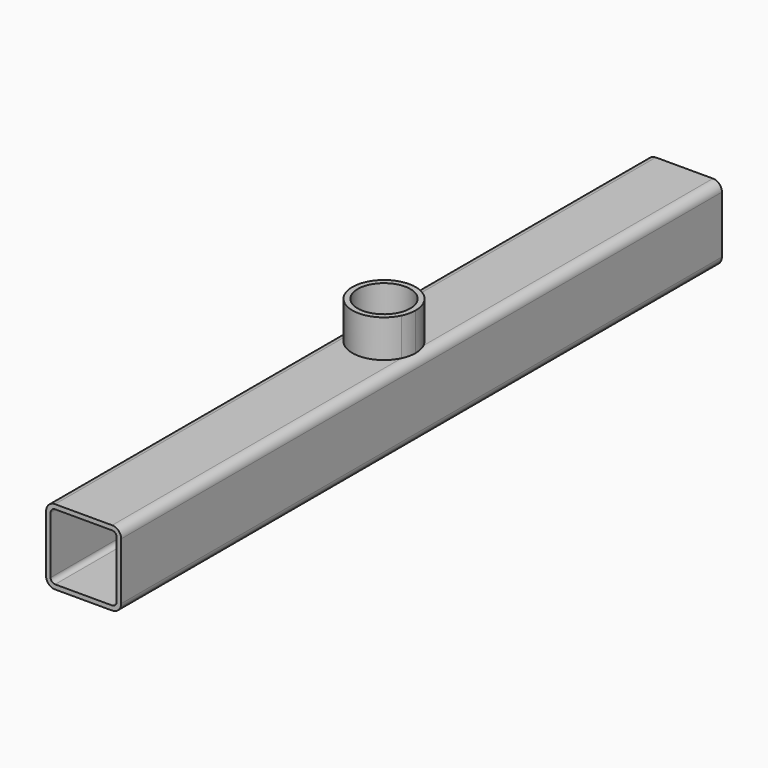
from build123d import *

# Parameters (mm, degrees)
F0_W     = 50
F0_H     = 50
F1_DEPTH = 500
F2_R     = 6
F3_T     = -3
F4_R     = 17.526
F5_DEPTH = 25


with BuildPart() as f1:
    # F0 (on Front) → F1 (new body)
    with BuildSketch(Plane.XZ):
        Rectangle(F0_W, F0_H)
    extrude(amount=F1_DEPTH)

    # F2
    f2_edges = [f1.edges().sort_by_distance(p)[0] for p in [
        (25, -250, 25),
        (-25, -250, 25),
        (25, -250, -25),
        (-25, -250, -25),
    ]]
    fillet(f2_edges, radius=F2_R)

    # F3
    f3_openings = [f1.faces().sort_by_distance(p)[0] for p in [
        (0, 0, 0),
        (0, -500, 0),
    ]]
    offset(amount=F3_T, openings=f3_openings)

    # F4 (on face) → F5 (join)
    with BuildSketch(Plane.XY.offset(25)):
        with BuildLine():
            ThreePointArc((19, -259.1351367806), (20.5549108974, -254.6846944404), (21.082, -250))
            ThreePointArc((21.082, -250), (20.5549108974, -245.3153055596), (19, -240.8648632194))
            Line((19, -240.8648632194), (19, -259.1351367806))
        make_face()
        with BuildLine():
            Line((19, -259.1351367806), (19, -240.8648632194))
            ThreePointArc((19, -240.8648632194), (0, -228.918), (-19, -240.8648632194))
            Line((-19, -240.8648632194), (-19, -259.1351367806))
            ThreePointArc((-19, -259.1351367806), (0, -271.082), (19, -259.1351367806))
        make_face()
        with Locations((0, -250)):
            Circle(F4_R, mode=Mode.SUBTRACT)
        with BuildLine():
            Line((-19, -259.1351367806), (-19, -240.8648632194))
            ThreePointArc((-19, -240.8648632194), (-21.082, -250), (-19, -259.1351367806))
        make_face()
    extrude(amount=F5_DEPTH)


solid = f1.part
